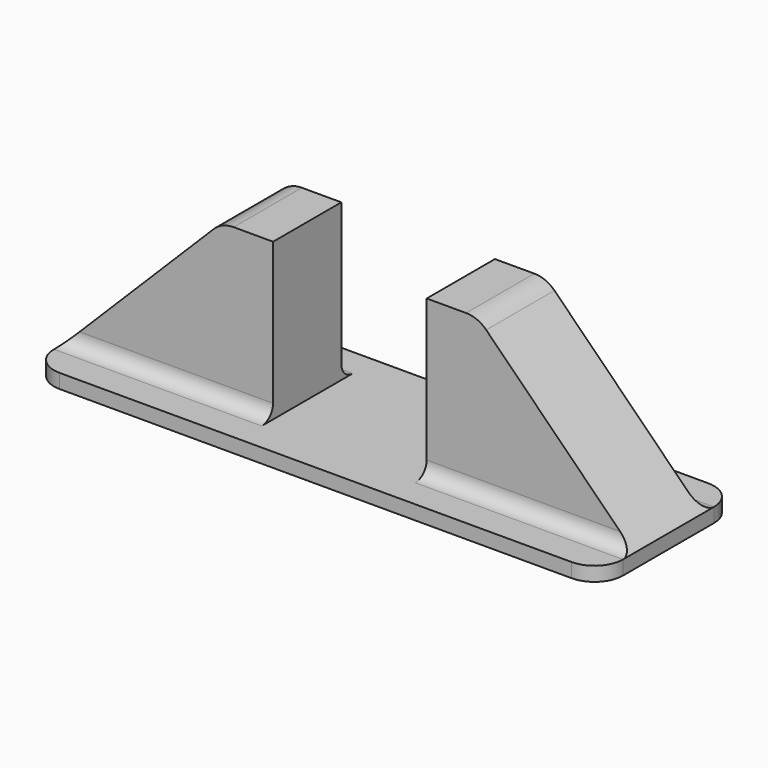
from build123d import *

# Parameters (mm, degrees)
F0_W         = 200
F0_H         = 30
F1_DEPTH     = 60
F2_SIZE      = 55
F3_SIZE      = 55
F4_W         = 54
F4_H         = 30
F5_DEPTH     = 55
F7_DEPTH     = 15
F8_R         = 10
F9_R         = 4.99999
F11_DEPTH    = 15
F12_T4_DEPTH = 73
F12_T9_DEPTH = 73
F13_R        = 10


# Not quite as in the source:
# - a fillet or chamfer that OpenCascade refuses, or shapes differently, is made with other operations: its cross-section is extruded or revolved along the edge and cut away or added
# - a fillet or chamfer is up to 0.001 mm smaller than in the source, because OpenCascade refuses the exact size


with BuildPart() as f1:
    # F0 (on Top) → F1 (new body)
    with BuildSketch(Plane.XY):
        with Locations((75.0721136101, 7.3799993843)):
            Rectangle(F0_W, F0_H)
    extrude(amount=F1_DEPTH)

    # F2
    f2_edges = [f1.edges().sort_by_distance(p)[0] for p in [
        (175.072114, 7.379999, 60),
    ]]
    chamfer(f2_edges, length=F2_SIZE)

    # F3
    f3_edges = [f1.edges().sort_by_distance(p)[0] for p in [
        (-24.927886, 7.379999, 60),
    ]]
    chamfer(f3_edges, length=F3_SIZE)

    # F4 (on face) → F5 (cut)
    with BuildSketch(Plane.XY.offset(60)):
        with Locations((75.0721136101, 7.3799993843)):
            Rectangle(F4_W, F4_H)
    extrude(amount=-F5_DEPTH, mode=Mode.SUBTRACT)

    # F6 (on face) → F7 (join)
    with BuildSketch(Plane.XZ.offset(7.6200006157)):
        Polygon((48.0721136101, 5), (-24.9278863899, 5), (-24.9278863899, 0), (175.0721136101, 0), (175.0721136101, 5), (102.0721136101, 5), align=None)
    extrude(amount=F7_DEPTH)

    # F8
    f8_edges = [f1.edges().sort_by_distance(p)[0] for p in [
        (175.072114, -22.620001, 2.5),
        (-24.927886, -22.620001, 2.5),
    ]]
    fillet(f8_edges, radius=F8_R)

    # F9 (radius 5 in the source; OpenCascade refuses exactly that, so slightly less here)
    f9_edges = [f1.edges().sort_by_distance(p)[0] for p in [
        (138.572114, -7.620001, 5),
        (11.572114, -7.620001, 5),
    ]]
    fillet(f9_edges, radius=F9_R)

    # F10 (on face) → F11 (join)
    with BuildSketch(Plane(origin=(0, 22.3799993843, 0), x_dir=(-1, 0, 0), z_dir=(0, 1, 0))):
        Polygon((-102.0721136101, 5), (-175.0721136101, 5), (-175.0721136101, 0), (24.9278863899, 0), (24.9278863899, 5), (-48.0721136101, 5), align=None)
    extrude(amount=F11_DEPTH)

    # F12: fillet of radius 5 on 2 edges, made by hand


with BuildPart() as f12_tool2:
    # F12_s3 → F12_t4 (new body)
    with BuildSketch(Plane.YZ.offset(102.0721136101)):
        with BuildLine():
            ThreePointArc((27.3799993843, 5), (23.8444654784, 6.4644660941), (22.3799993843, 10))
            Line((22.3799993843, 10), (22.3799993843, 5))
            Line((22.3799993843, 5), (27.3799993843, 5))
        make_face()
    extrude(amount=F12_T4_DEPTH)

    split(bisect_by=Plane(origin=(90.0360568051, 0, 90.0360568051), x_dir=(0, 1, 0), z_dir=(-0.7071067812, 0, -0.7071067812)), keep=Keep.TOP)


with BuildPart() as f1_1:
    add(f1.part)

    # F12_t1: union F12_tool2
    add(f12_tool2.part)


with BuildPart() as f12_tool7:
    # F12_s8 → F12_t9 (new body)
    with BuildSketch(Plane.YZ.offset(-24.9278863899)):
        with BuildLine():
            ThreePointArc((27.3799993843, 5), (23.8444654784, 6.4644660941), (22.3799993843, 10))
            Line((22.3799993843, 10), (22.3799993843, 5))
            Line((22.3799993843, 5), (27.3799993843, 5))
        make_face()
    extrude(amount=F12_T9_DEPTH)

    split(bisect_by=Plane(origin=(-14.9639431949, 0, 14.9639431949), x_dir=(0, 1, 0), z_dir=(0.7071067812, 0, -0.7071067812)), keep=Keep.TOP)


with BuildPart() as f1_2:
    add(f1_1.part)

    # F12_t6: union F12_tool7
    add(f12_tool7.part)

    # F13
    f13_edges = [f1_2.edges().sort_by_distance(p)[0] for p in [
        (175.072114, 37.379999, 2.5),
        (-24.927886, 37.379999, 2.5),
        (120.072114, 7.379999, 60),
        (30.072114, 7.379999, 60),
    ]]
    fillet(f13_edges, radius=F13_R)


solid = f1_2.part
